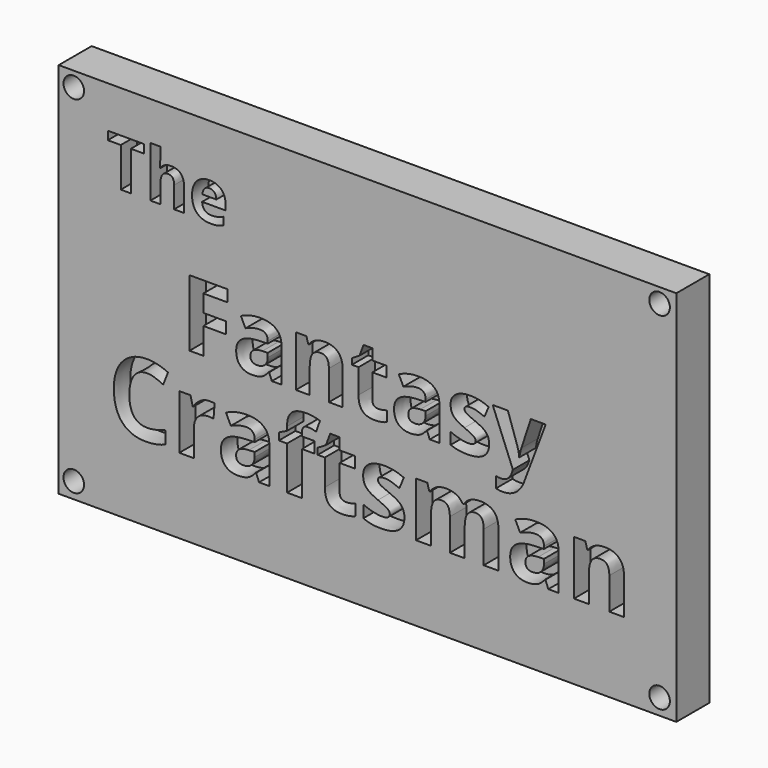
from build123d import *

# Parameters (mm, degrees)
F0_W         = 150
F0_H         = 91.6490518779
F1_DEPTH     = 10
F6_D         = 5
F2_TEXT_SIZE = 16.2258091777
F3_TEXT_SIZE = 22.6183931517
F4_TEXT_SIZE = 24.1902139452
F7_DEPTH     = 5


# Not quite as in the source:
# - Text() gives the source's letters only with a copy of the font that has no kerning and outlines rounded to 1/6400 em; it was checked with that copy


with BuildPart() as f1:
    # F0 (on Front) → F1 (new body)
    with BuildSketch(Plane.XZ):
        with Locations((1.0429620743, 10.1316198707)):
            Rectangle(F0_W, F0_H)
    extrude(amount=F1_DEPTH)

    # F6 (through all)
    with Locations(Plane.XZ.offset(10)):
        with Locations((-70.2991038561, 52.4036735296), (-70.2991038561, -31.7973382771), (71.9715729356, 52.4036735296), (71.9715729356, -31.7973382771)):
            Hole(F6_D / 2)

    # F2 (on face) + F3 (on face) + F4 (on face) → F7 (cut)
    with BuildSketch(Plane.XZ.offset(10)):
        with Locations((-62.3585847461, 34.2297949761)):
            Text('The', F2_TEXT_SIZE, font='Open Sans', font_style=FontStyle.BOLD, text_align=(TextAlign.LEFT, TextAlign.BOTTOM))
    with BuildSketch(Plane.XZ.offset(10)):
        with Locations((-44.2229185299, 5.224484421)):
            Text('Fantasy', F3_TEXT_SIZE, font='Open Sans', font_style=FontStyle.BOLD, text_align=(TextAlign.LEFT, TextAlign.BOTTOM))
    with BuildSketch(Plane.XZ.offset(10)):
        with Locations((-61.9800202549, -17.4169540405)):
            Text('Craftsman', F4_TEXT_SIZE, font='Open Sans', font_style=FontStyle.BOLD, text_align=(TextAlign.LEFT, TextAlign.BOTTOM))
    extrude(amount=-F7_DEPTH, mode=Mode.SUBTRACT)


solid = f1.part
